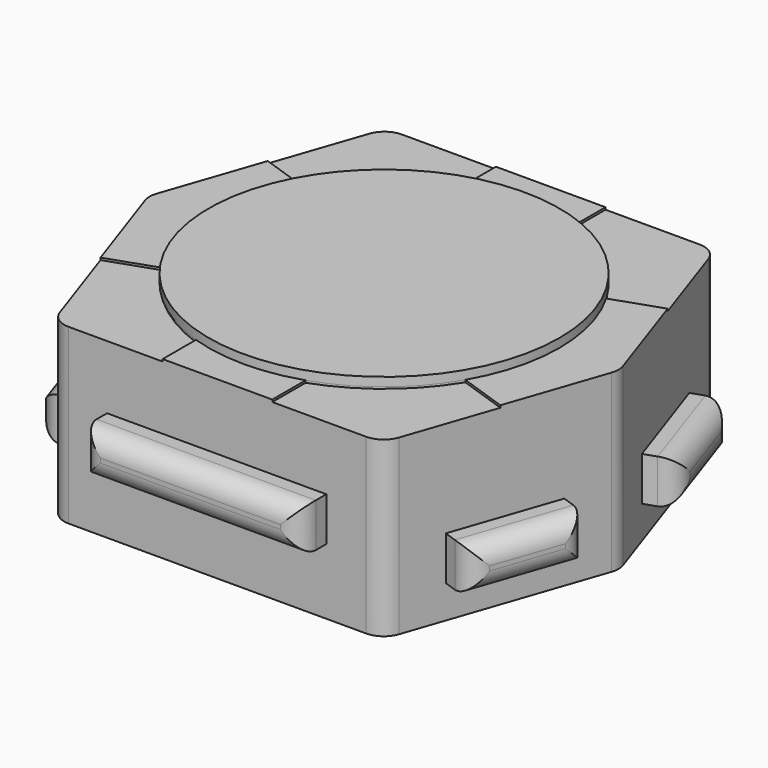
from build123d import *

# Parameters (mm, degrees)
F1_DEPTH  = 80
F4_R      = 80
F5_DEPTH  = 4
F7_DEPTH  = 50
F8_R      = 65
F9_DEPTH  = 25
F11_DEPTH = 1
F13_R     = 10
F15_W     = 50
F15_H     = 20
F16_DEPTH = 15
F14_W     = 50
F14_H     = 20
F17_DEPTH = 15
F18_W     = 50
F18_H     = 20
F19_DEPTH = 15
F20_W     = 50
F20_H     = 20
F21_DEPTH = 15
F22_W     = 100
F22_H     = 20
F23_DEPTH = 15
F24_W     = 100
F24_H     = 20
F25_DEPTH = 15
F26_R     = 9
F26_2_R   = 9
F26_3_R   = 9
F26_4_R   = 9
F26_5_R   = 9
F26_6_R   = 9


# Not quite as in the source:
# - the program builds the solid bodies; features that only make, move or delete a surface that nothing else refers to are left out


with BuildPart() as f1:
    # F0 (on Top) → F1 (new body)
    with BuildSketch(Plane.XY):
        Polygon((75, 95), (0, 95), (0, 0), (107.5, 0), align=None)
        Polygon((0, 0), (0, 95), (-75, 95), (-107.5, 0), align=None)
        Polygon((107.5, 0), (0, 0), (0, -95), (75, -95), align=None)
        Polygon((0, -95), (0, 0), (-107.5, 0), (-75, -95), align=None)
    extrude(amount=F1_DEPTH)

    # F4 (on face) → F5 (join)
    with BuildSketch(Plane.XY.offset(80)):
        Circle(F4_R)
    extrude(amount=F5_DEPTH)

    # F6 (on face) → F7 (cut)
    with BuildSketch(Plane(origin=(0, 0, 0), x_dir=(1, 0, 0), z_dir=(0, 0, -1))):
        Polygon((67.8520601958, 85), (-67.8520601958, 85), (-96.9310075642, 0), (-67.8520601958, -85), (67.8520601958, -85), (96.9310075642, 0), align=None)
    extrude(amount=-F7_DEPTH, mode=Mode.SUBTRACT)

    # F8 (on face) → F9 (cut)
    with BuildSketch(Plane(origin=(0, 0, 50), x_dir=(1, 0, 0), z_dir=(0, 0, -1))):
        Circle(F8_R)
    extrude(amount=-F9_DEPTH, mode=Mode.SUBTRACT)

    # F10 (on face) → F11 (cut)
    with BuildSketch(Plane.XY.offset(80)):
        with BuildLine():
            Line((25, -95), (75, -95))
            Line((75, -95), (91.1843839531, -47.6918007523))
            Line((91.1843839531, -47.6918007523), (69.1859204708, -40.1660106136))
            ThreePointArc((69.1859204708, -40.1660106136), (50.1602708255, -61.8626277464), (25, -75.9934207679))
            Line((25, -75.9934207679), (25, -95))
        make_face()
        with BuildLine():
            Line((91.1843839531, 47.6918007523), (75, 95))
            Line((75, 95), (25, 95))
            Line((25, 95), (25, 75.9934207679))
            ThreePointArc((25, 75.9934207679), (50.1602708255, 61.8626277464), (69.1859204708, 40.1660106136))
            Line((69.1859204708, 40.1660106136), (91.1843839531, 47.6918007523))
        make_face()
        with BuildLine():
            Line((-25, 95), (-75, 95))
            Line((-75, 95), (-91.1843839531, 47.6918007523))
            Line((-91.1843839531, 47.6918007523), (-69.1859204708, 40.1660106136))
            ThreePointArc((-69.1859204708, 40.1660106136), (-50.1602708255, 61.8626277464), (-25, 75.9934207679))
            Line((-25, 75.9934207679), (-25, 95))
        make_face()
        with BuildLine():
            ThreePointArc((-25, -75.9934207679), (-50.1602708255, -61.8626277464), (-69.1859204708, -40.1660106136))
            Line((-69.1859204708, -40.1660106136), (-91.1843839531, -47.6918007523))
            Line((-91.1843839531, -47.6918007523), (-75, -95))
            Line((-75, -95), (-25, -95))
            Line((-25, -95), (-25, -75.9934207679))
        make_face()
    extrude(amount=-F11_DEPTH, mode=Mode.SUBTRACT)

    # F13
    f13_edges = [f1.edges().sort_by_distance(p)[0] for p in [
        (-75, -95, 39.5),
        (75, -95, 39.5),
        (107.5, 0, 40),
        (75, 95, 39.5),
        (-75, 95, 39.5),
        (-107.5, 0, 40),
    ]]
    fillet(f13_edges, radius=F13_R)


with BuildPart() as f16:
    # F15 (on face) → F16 (new body)
    with BuildSketch(Plane(origin=(-96.2368257905, 32.9231246125, 0), x_dir=(-0.3236876791, -0.946163985, 0), z_dir=(-0.946163985, 0.3236876791, 0))):
        with Locations((-13.6246271323, 25)):
            Rectangle(F15_W, F15_H)
    extrude(amount=F16_DEPTH)

    # F26#4
    f26_4_edges = [f16.edges().sort_by_distance(p)[0] for p in [
        (-114.111354, 27.015472, 25),
        (-106.019162, 50.669571, 35),
        (-97.92697, 74.323671, 25),
        (-106.019162, 50.669571, 15),
    ]]
    fillet(f26_4_edges, radius=F26_4_R)


with BuildPart() as f17:
    # F14 (on face) → F17 (new body)
    with BuildSketch(Plane(origin=(-96.2368257905, -32.9231246125, 0), x_dir=(0.3236876791, -0.946163985, 0), z_dir=(-0.946163985, -0.3236876791, 0))):
        with Locations((13.6246271323, 25)):
            Rectangle(F14_W, F14_H)
    extrude(amount=F17_DEPTH)

    # F26#3
    f26_3_edges = [f17.edges().sort_by_distance(p)[0] for p in [
        (-106.019162, -50.669571, 35),
        (-97.92697, -74.323671, 25),
        (-106.019162, -50.669571, 15),
        (-114.111354, -27.015472, 25),
    ]]
    fillet(f26_3_edges, radius=F26_3_R)


with BuildPart() as f19:
    # F18 (on face) → F19 (new body)
    with BuildSketch(Plane(origin=(96.2368257905, 32.9231246125, 0), x_dir=(-0.3236876791, 0.946163985, 0), z_dir=(0.946163985, 0.3236876791, 0))):
        with Locations((13.4610628366, 25)):
            Rectangle(F18_W, F18_H)
    extrude(amount=F19_DEPTH)

    # F26#2
    f26_2_edges = [f19.edges().sort_by_distance(p)[0] for p in [
        (106.072105, 50.514813, 35),
        (114.164297, 26.860713, 25),
        (106.072105, 50.514813, 15),
        (97.979913, 74.168912, 25),
    ]]
    fillet(f26_2_edges, radius=F26_2_R)


with BuildPart() as f21:
    # F20 (on face) → F21 (new body)
    with BuildSketch(Plane(origin=(96.2368257905, -32.9231246125, 0), x_dir=(0.3236876791, 0.946163985, 0), z_dir=(0.946163985, -0.3236876791, 0))):
        with Locations((-13.6246271323, 25)):
            Rectangle(F20_W, F20_H)
    extrude(amount=F21_DEPTH)

    # F26
    f26_edges = [f21.edges().sort_by_distance(p)[0] for p in [
        (106.019162, -50.669571, 35),
        (97.92697, -74.323671, 25),
        (106.019162, -50.669571, 15),
        (114.111354, -27.015472, 25),
    ]]
    fillet(f26_edges, radius=F26_R)


with BuildPart() as f23:
    # F22 (on face) → F23 (new body)
    with BuildSketch(Plane(origin=(0, 95, 0), x_dir=(-1, 0, 0), z_dir=(0, 1, 0))):
        with Locations((-0.3520601958, 40)):
            Rectangle(F22_W, F22_H)
    extrude(amount=F23_DEPTH)

    # F26#5
    f26_5_edges = [f23.edges().sort_by_distance(p)[0] for p in [
        (0.35206, 110, 50),
        (50.35206, 110, 40),
        (0.35206, 110, 30),
        (-49.64794, 110, 40),
    ]]
    fillet(f26_5_edges, radius=F26_5_R)


with BuildPart() as f25:
    # F24 (on face) → F25 (new body)
    with BuildSketch(Plane.XZ.offset(95)):
        with Locations((-0.3520601958, 40)):
            Rectangle(F24_W, F24_H)
    extrude(amount=F25_DEPTH)

    # F26#6
    f26_6_edges = [f25.edges().sort_by_distance(p)[0] for p in [
        (-0.35206, -110, 30),
        (49.64794, -110, 40),
        (-0.35206, -110, 50),
        (-50.35206, -110, 40),
    ]]
    fillet(f26_6_edges, radius=F26_6_R)


solid = Compound([f1.part, f16.part, f17.part, f19.part, f21.part, f23.part, f25.part])
